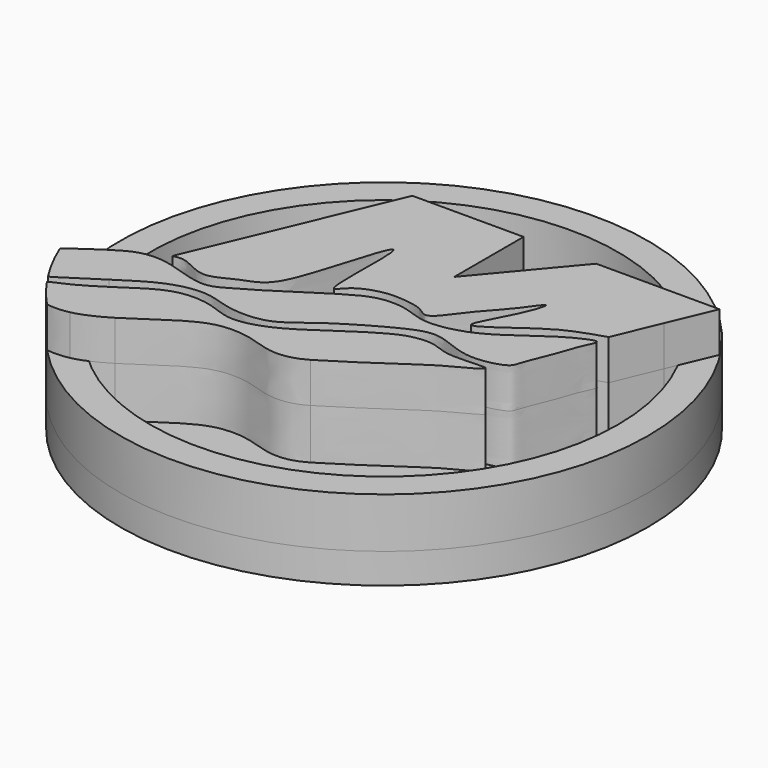
from build123d import *

# Parameters (mm, degrees)
F1_DEPTH = 5
F3_R     = 26.2887406731
F4_DEPTH = 3
F5_R     = 26.2887406731
F5_R_2   = 23.2887406731
F6_DEPTH = 5
F7_DEPTH = 4


# Not quite as in the source:
# - the program builds the solid bodies; features that only make, move or delete a surface that nothing else refers to are left out


with BuildPart() as f1:
    # F0 (on Top) → F1 (new body)
    with BuildSketch(Plane.XY):
        with BuildLine():
            Line((23.7963441759, 15.1072172448), (19.2888453603, 15.1072172448))
            Line((19.2888453603, 15.1072172448), (15.7133191824, 15.1072172448))
            Line((15.7133191824, 15.1072172448), (8.4771029651, 6.4736609347))
            Line((8.4771029651, 6.4736609347), (8.4771029651, 15.1072172448))
            Line((8.4771029651, 15.1072172448), (-2.6017946657, 15.1072172448))
            Line((-2.6017946657, 15.1072172448), (-10.8361104503, -4.4555221684))
            add(Edge.make_bspline(
                [(-10.8361104503, -4.4555221684), (-10.4343693569, -4.3826211181), (-9.4633807702, -4.2064228428), (-7.0519921591, -5.9650430703), (-4.5816475592, -4.2933295263), (-1.9676882693, -3.6963901633), (-0.348217337, 0.2336616175), (2.8072826499, 12.0532678023), (1.722219715, -2.4735248895), (3.2704441394, 0.2714703564), (5.9007571837, 1.1160671049), (7.6100584737, 1.0695083777), (9.7606046095, 0.80719369), (10.9998631376, -0.5516776232), (13.1006310402, 2.8030409274), (15.4310289621, 5.0140619141), (17.5091121303, 8.2744638424), (16.3904741823, 4.5851540219), (13.0723392276, -0.6340270806), (18.3789070792, 3.4320853925), (20.9677968345, 5.0346125934), (23.1353828408, 5.7286832434), (24.1836215662, 6.0643339311)],
                knots=[0, 0, 0, 0, 0.0327510511, 0.0791576898, 0.1263933458, 0.1702012891, 0.2344891078, 0.3072025778, 0.3877226152, 0.4179882815, 0.4668096706, 0.505355151, 0.5469692057, 0.5791355047, 0.6303999864, 0.6879051425, 0.7309066345, 0.7774447, 0.8355858799, 0.8933134939, 0.9484066944, 1, 1, 1, 1], degree=3))
            Line((24.1836215662, 6.0643339311), (26.0867792794, 10.5857755879))
            Line((26.0867792794, 10.5857755879), (27.9899369925, 15.1072172448))
            Line((27.9899369925, 15.1072172448), (23.7963441759, 15.1072172448))
        make_face()
    extrude(amount=F1_DEPTH)


with BuildPart() as f1b:
    # F0 (on Top) → F1, piece 2 (new body)
    with BuildSketch(Plane.XY):
        with BuildLine():
            add(Edge.make_bspline(
                [(-14.2682872836, -6.1061690629), (-13.9583456939, -5.944462994), (-12.8429352258, -5.448382868), (-10.9860167046, -5.412374749), (-9.1787939742, -5.9127964853), (-5.9793578204, -7.0172917936), (-4.0433647011, -5.9630021206), (-1.5211815589, -4.4928677724), (0.7975745464, -2.9155490623), (3.9581349912, -0.9138991304), (6.1675128346, 0.1685962635), (8.8795683569, 0.0979966698), (10.7340686313, -0.8299048946), (13.1390384474, -0.7787582686), (15.9695425229, 0.1150245467), (18.7167386382, 1.9965785265), (21.3963592711, 3.9886145718), (24.4717261058, 5.3972223641), (23.407577476, 3.5636539698), (22.7520616494, 1.238886965), (21.5384075596, -1.4414293553), (21.3931156013, -2.5647004359), (19.2322081343, -3.25961114), (16.6192257522, -3.2651965894), (13.5696174174, -1.586565479), (10.6893269067, -2.777644785), (7.5559143837, -4.5256417888), (4.4396788093, -6.5161939366), (1.9611343286, -8.7458099538), (-1.9411777654, -8.6892226306), (-4.0847560172, -7.7755478782), (-6.3092965475, -7.7244280444), (-9.0898670503, -8.5929852237), (-11.0554204683, -9.9125631023), (-12.1913468016, -10.6487929135), (-12.1952494823, -10.6513220777)],
                knots=[0.0967557357, 0.0967557357, 0.0967557357, 0.0967557357, 0.1059408277, 0.1294460595, 0.1510625476, 0.1786405627, 0.2011593113, 0.2272611402, 0.253723758, 0.2834993747, 0.3079027085, 0.332608255, 0.3547046452, 0.378165643, 0.4046956115, 0.4328058229, 0.4629056021, 0.4863360462, 0.5029567511, 0.5286947841, 0.5550250628, 0.5703774393, 0.5921342915, 0.6175623632, 0.6454177535, 0.671755873, 0.7012996512, 0.7311226102, 0.7590522215, 0.7886195648, 0.8122261167, 0.8346470578, 0.8606740928, 0.8907909111, 0.890894715, 0.890894715, 0.890894715, 0.890894715], degree=3))
            add(Edge.make_bspline(
                [(-14.2682872836, -6.1061690629), (-13.763419632, -7.5022555749), (-13.0535168829, -9.1852694628), (-12.1952494823, -10.6513220777)],
                knots=[0.4139602767, 0.4139602767, 0.4139602767, 0.4139602767, 0.4587948897, 0.4587948897, 0.4587948897, 0.4587948897], degree=3))
        make_face()
        with BuildLine():
            add(Edge.make_bspline(
                [(-18.4733406444, -8.9109834623), (-18.4225927781, -8.8727345044), (-17.5949119208, -8.2505417581), (-16.3246093096, -7.4049949505), (-14.8757612608, -6.4231069379), (-14.2682872836, -6.1061690629)],
                knots=[0.0511774027, 0.0511774027, 0.0511774027, 0.0511774027, 0.0528592406, 0.0787532973, 0.0967557357, 0.0967557357, 0.0967557357, 0.0967557357], degree=3))
            ThreePointArc((-18.4733406444, -8.9109834623), (-17.4533098383, -11.1220400627), (-16.233074702, -13.2292325901))
            add(Edge.make_bspline(
                [(-12.1952494823, -10.6513220777), (-13.3084581911, -11.372746103), (-15.0519652777, -12.4684214036), (-15.9187131878, -13.0770255012), (-16.233074702, -13.2292325901)],
                knots=[0.890894715, 0.890894715, 0.890894715, 0.890894715, 0.9205039546, 0.9343419902, 0.9343419902, 0.9343419902, 0.9343419902], degree=3))
            add(Edge.make_bspline(
                [(-14.2682872836, -6.1061690629), (-13.763419632, -7.5022555749), (-13.0535168829, -9.1852694628), (-12.1952494823, -10.6513220777)],
                knots=[0.4139602767, 0.4139602767, 0.4139602767, 0.4139602767, 0.4587948897, 0.4587948897, 0.4587948897, 0.4587948897], degree=3))
        make_face()
    extrude(amount=F1_DEPTH)


with BuildPart() as f1c:
    # F0 (on Top) → F1, piece 3 (new body)
    with BuildSketch(Plane.XY):
        with BuildLine():
            add(Edge.make_bspline(
                [(-15.7605147548, -13.9389334253), (-15.3406636143, -13.7657247702), (-13.8987388774, -13.1354481012), (-12.5504908967, -12.3350365424), (-11.543254048, -11.6757772259)],
                knots=[0.0354513148, 0.0354513148, 0.0354513148, 0.0354513148, 0.0603306484, 0.1218229664, 0.1218229664, 0.1218229664, 0.1218229664], degree=3))
            ThreePointArc((-15.7605147548, -13.9389334253), (-14.6172697034, -15.4741917012), (-13.3653424335, -16.9221921612))
            add(Edge.make_bspline(
                [(-11.1533682793, -16.8522614986), (-11.8840144876, -17.0094130762), (-12.6325177474, -17.0403801326), (-13.3653424335, -16.9221921612)],
                knots=[0.7630377841, 0.7630377841, 0.7630377841, 0.7630377841, 0.8411046366, 0.8411046366, 0.8411046366, 0.8411046366], degree=3))
            add(Edge.make_bspline(
                [(-7.8308843323, -15.3918337734), (-8.9366307934, -16.0646229924), (-10.0236542222, -16.6092761189), (-11.1533682793, -16.8522614986)],
                knots=[0.6423320039, 0.6423320039, 0.6423320039, 0.6423320039, 0.7630377841, 0.7630377841, 0.7630377841, 0.7630377841], degree=3))
            add(Edge.make_bspline(
                [(-11.5432540569, -11.675777213), (-10.5062143739, -13.1668444028), (-9.2924766715, -14.2922474657), (-7.8308843323, -15.3918337734)],
                knots=[0.4697029588, 0.4697029588, 0.4697029588, 0.4697029588, 0.5198308803, 0.5198308803, 0.5198308803, 0.5198308803], degree=3))
        make_face()
        with BuildLine():
            add(Edge.make_bspline(
                [(-11.543254048, -11.6757772259), (-10.4938395857, -10.9889117067), (-8.4854155983, -9.5586653969), (-6.0626847181, -8.7152044134), (-3.2423122223, -8.9241669329), (-0.8827377625, -10.2079591044), (3.103680717, -9.1322896947), (6.8496872557, -6.3813414206), (10.5054561575, -4.0470436384), (12.2531442064, -3.3835340931), (14.4546368111, -3.1935687837), (16.1394384372, -4.335398428), (21.7293278697, -3.4728690921), (17.0357980083, -5.6999809216), (15.0975423786, -7.1088768473), (10.7528156625, -10.0273475201), (9.1526531106, -11.0068103937), (8.4771029651, -11.4203160629)],
                knots=[0.1218229664, 0.1218229664, 0.1218229664, 0.1218229664, 0.1858902489, 0.2387130203, 0.292978794, 0.3460486821, 0.4108545688, 0.4843417303, 0.5527701287, 0.5980255452, 0.6441533068, 0.6949374354, 0.7565105586, 0.8126883461, 0.8712297744, 0.9456365894, 1, 1, 1, 1], degree=3))
            add(Edge.make_bspline(
                [(-11.5432540569, -11.675777213), (-10.5062143739, -13.1668444028), (-9.2924766715, -14.2922474657), (-7.8308843323, -15.3918337734)],
                knots=[0.4697029588, 0.4697029588, 0.4697029588, 0.4697029588, 0.5198308803, 0.5198308803, 0.5198308803, 0.5198308803], degree=3))
            add(Edge.make_bspline(
                [(8.4771029651, -11.4203160629), (8.0580429463, -11.6423110517), (7.1320411504, -12.1328504444), (4.8515297092, -12.3324551861), (2.3223342989, -11.2238723354), (-1.1203404944, -11.12165998), (-4.2687677404, -12.9577305352), (-6.6215137336, -14.6559946554), (-7.8308843323, -15.3918337734)],
                knots=[0, 0, 0, 0, 0.0770619252, 0.1702855388, 0.275538346, 0.3901707876, 0.5103143789, 0.6423320039, 0.6423320039, 0.6423320039, 0.6423320039], degree=3))
        make_face()
    extrude(amount=F1_DEPTH)


with BuildPart() as f4:
    # F3 (on face) → F4 (new body)
    with BuildSketch(Plane(origin=(0, 0, 0), x_dir=(1, 0, 0), z_dir=(0, 0, -1))):
        with Locations((5.8820461854, -0.9841172723)):
            Circle(F3_R)
    extrude(amount=F4_DEPTH)


with BuildPart() as f6:
    # F5 (on face) → F6 (new body, through all)
    with BuildSketch(Plane.XY.offset(5)):
        with Locations((5.8820461854, 0.9841172723)):
            Circle(F5_R)
        with Locations((5.8820461854, 0.9841172723)):
            Circle(F5_R_2, mode=Mode.SUBTRACT)
    extrude(amount=-F6_DEPTH)


with BuildPart() as f7:
    # F7 (new): a face of the model
    f7_faces = [f1.part.faces().sort_by_distance(p)[0] for p in [
        (7.382294917, 7.0109600974, 5),
    ]]
    extrude(f7_faces, amount=F7_DEPTH)


with BuildPart() as f7b:
    # F7#2 (new): a face of the model
    f7_2_faces = [f1b.part.faces().sort_by_distance(p)[0] for p in [
        (2.5605354423, -4.4747167723, 5),
    ]]
    extrude(f7_2_faces, amount=F7_DEPTH)


with BuildPart() as f7c:
    # F7#3 (new): a face of the model
    f7_3_faces = [f1c.part.faces().sort_by_distance(p)[0] for p in [
        (1.331537316, -10.0293950589, 5),
    ]]
    extrude(f7_3_faces, amount=F7_DEPTH)


solid = Compound([f1.part, f1b.part, f1c.part, f4.part, f6.part, f7.part, f7b.part, f7c.part])
